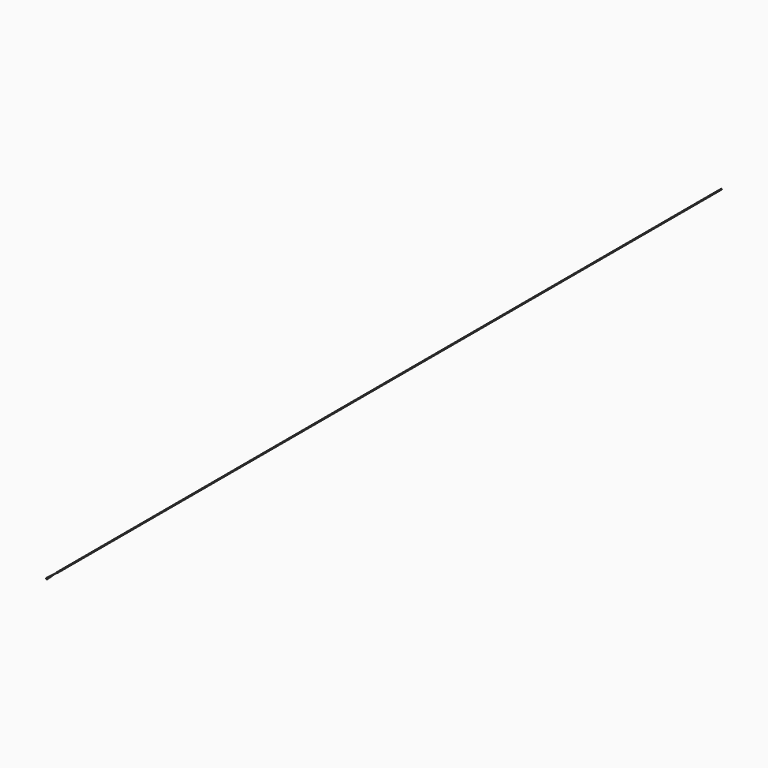
from build123d import *

# Parameters (mm, degrees)
F2_R      = 0.0625
F7_DEPTH  = 0.2
F4_R      = 0.0625
F8_DEPTH  = 0.3
F6_R      = 0.0625
F9_DEPTH  = 349.35
F11_R     = 0.1875
F11_R_2   = 0.0625
F12_DEPTH = 349


# Not quite as in the source:
# - a feature names something its author has since deleted; it is built from what else it names


with BuildPart() as f7:
    # F2 (on offset) → F7 (new body)
    with BuildSketch(Plane.XZ.offset(-0.15)):
        Circle(F2_R)
    extrude(amount=-F7_DEPTH)


with BuildPart() as f8:
    # F4 (on offset) → F8 (new body)
    with BuildSketch(Plane.XZ.offset(-0.35)):
        Circle(F4_R)
    extrude(amount=-F8_DEPTH)


with BuildPart() as f9:
    # F6 (on offset) → F9 (new body)
    with BuildSketch(Plane.XZ.offset(-0.65)):
        Circle(F6_R)
    extrude(amount=-F9_DEPTH)


with BuildPart() as f12:
    # F11 (on offset) → F12 (new body)
    with BuildSketch(Plane.XZ.offset(-1)):
        Circle(F11_R)
        Circle(F11_R_2, mode=Mode.SUBTRACT)
    extrude(amount=-F12_DEPTH)


with BuildPart() as f14:
    # F13 (on Right) → F14 (revolve)
    with BuildSketch(Plane.YZ):
        with BuildLine():
            Line((-4.35, 0), (0.65, 0))
            Line((0.65, 0), (0.3491367389, 0.0277561471))
            add(Edge.make_bspline(
                [(0.3491367389, 0.0277561471), (0.3021492431, 0.0329769782), (0.2240491251, 0.0405844807), (0.2038690727, 0.0459227485), (0.1578124079, 0.0479448684)],
                knots=[0, 0, 0, 0, 0.5530440475, 1, 1, 1, 1], degree=3))
            Line((0.1578124079, 0.0479448684), (-4.35, 0.3))
            Line((-4.35, 0.3), (-4.35, 0))
        make_face()
    revolve(axis=Axis((0, -1.85, 0), (0, -1, 0)))


solid = Compound([f7.part, f8.part, f9.part, f12.part, f14.part])
